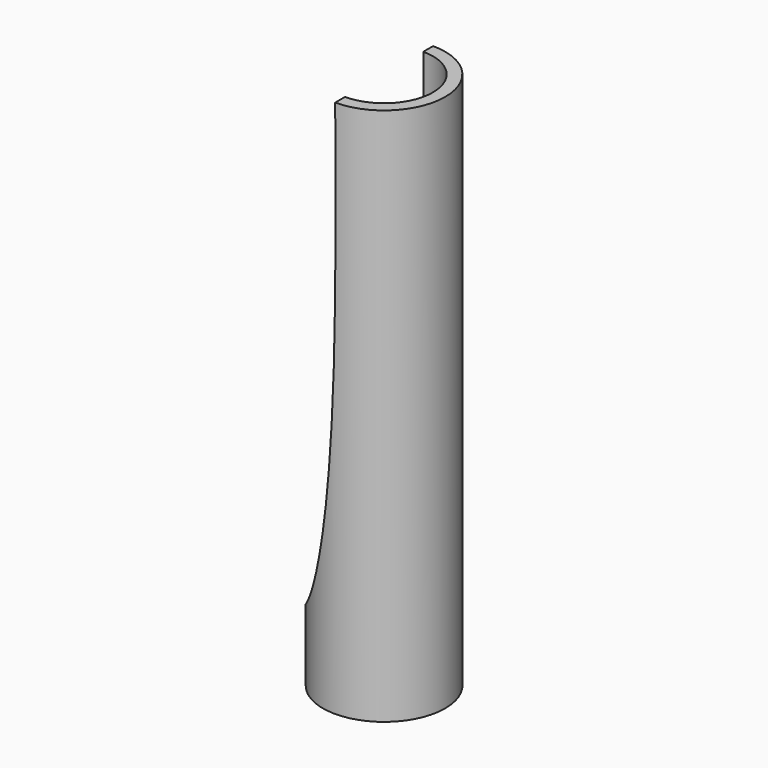
from build123d import *

# Parameters (mm, degrees)
F0_R          = 31.75
F0_R_2        = 25.4
F1_DEPTH      = 279.4
F3_DEPTH      = 31.751
F3_DEPTH_BACK = 31.751


with BuildPart() as f1:
    # F0 (on Top) → F1 (new body)
    with BuildSketch(Plane.XY):
        Circle(F0_R)
        Circle(F0_R_2, mode=Mode.SUBTRACT)
    extrude(amount=F1_DEPTH)

    # F2 (on Front) → F3 (cut, two sides)
    with BuildSketch(Plane.XZ) as f3_sk:
        with BuildLine():
            add(Edge.make_bspline(
                [(0, 298.2918024063), (0, 213.7468606234), (5.0540628254, 23.6161296496), (-40.6106183642, 33.05023015), (-57.3497712612, 12.2780762613)],
                knots=[0, 0, 0, 0, 0.685028541, 1, 1, 1, 1], degree=3))
            Line((0, 298.2918024063), (-57.3497712612, 299.4403541088))
            Line((-57.3497712612, 299.4403541088), (-57.3497712612, 12.2780762613))
        make_face()
    extrude(amount=F3_DEPTH, mode=Mode.SUBTRACT)
    extrude(f3_sk.sketch, amount=-F3_DEPTH_BACK, mode=Mode.SUBTRACT)


solid = f1.part
